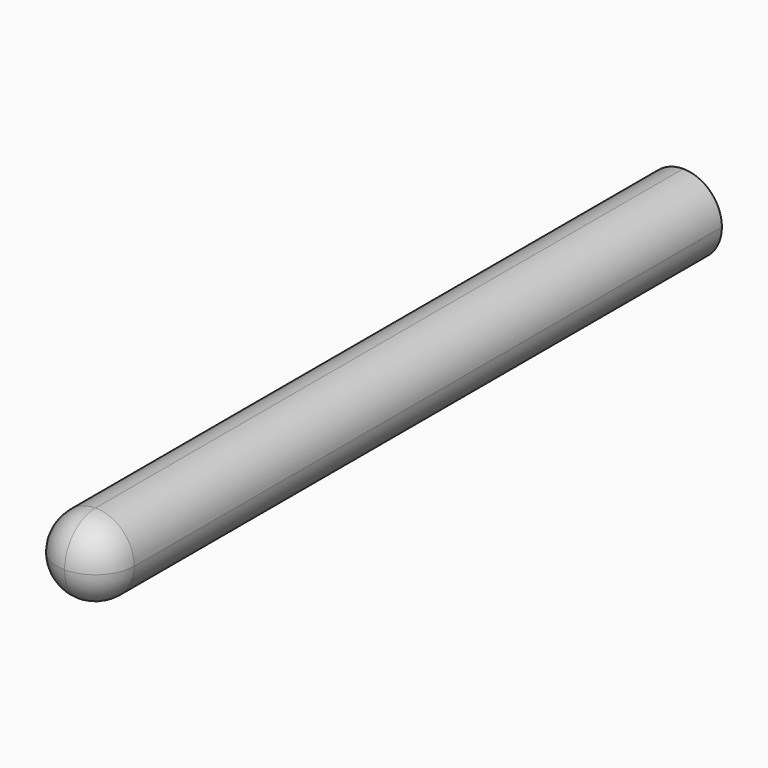
from build123d import *

# Parameters (mm, degrees)
F0_W     = 10
F0_H     = 10
F1_DEPTH = 100
F2_R     = 4.99999
F3_R     = 4.99999


# Not quite as in the source:
# - a fillet or chamfer is up to 0.001 mm smaller than in the source, because OpenCascade refuses the exact size


with BuildPart() as f1:
    # F0 (on Front) → F1 (new body)
    with BuildSketch(Plane.XZ):
        with Locations((-105.608215639, 32.9564241692)):
            Rectangle(F0_W, F0_H)
    extrude(amount=F1_DEPTH)

    # F2 (radius 5 in the source; OpenCascade refuses exactly that, so slightly less here)
    f2_edges = [f1.edges().sort_by_distance(p)[0] for p in [
        (-110.608216, -50, 37.956424),
        (-100.608216, -50, 37.956424),
        (-100.608216, -50, 27.956424),
        (-110.608216, -50, 27.956424),
    ]]
    fillet(f2_edges, radius=F2_R)

    # F3 (radius 5 in the source; OpenCascade refuses exactly that, so slightly less here)
    f3_edges = [f1.edges().sort_by_distance(p)[0] for p in [
        (-109.143752, -100, 36.491961),
    ]]
    fillet(f3_edges, radius=F3_R)


solid = f1.part
